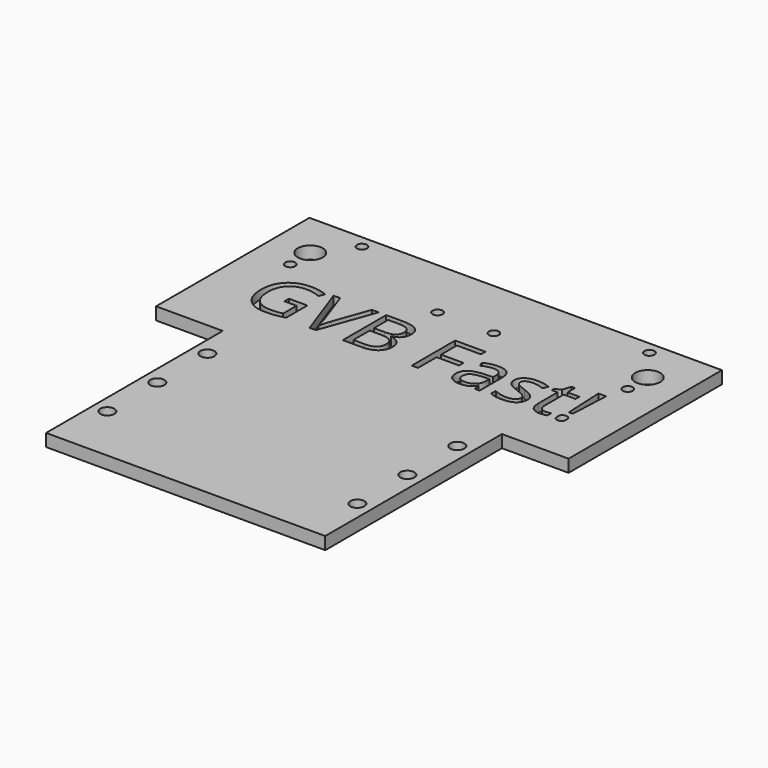
from build123d import *

# Parameters (mm, degrees)
F0_R         = 1.7
F0_R_2       = 1.2
F0_R_3       = 3
F1_DEPTH     = 3
F3_TEXT_SIZE = 18.2238832532
F4_DEPTH     = 2


# Not quite as in the source:
# - Text() gives the source's letters only with a copy of the font that has no kerning and outlines rounded to 1/6400 em; it was checked with that copy


with BuildPart() as f1:
    # F0 (on Top) → F1 (new body)
    with BuildSketch(Plane.XY):
        Polygon((0, 52.7634354346), (-49.5, 52.7634354346), (-49.5, 6.7634354346), (-33.5, 6.7634354346), (-33.5, -46.2365645654), (0, -46.2365645654), (33.5, -46.2365645654), (33.5, 6.7634354346), (49.5, 6.7634354346), (49.5, 52.7634354346), align=None)
        with Locations((-30, -32.2365645654)):
            Circle(F0_R, mode=Mode.SUBTRACT)
        with Locations((-30, -17.2365645654)):
            Circle(F0_R, mode=Mode.SUBTRACT)
        with Locations((-30, -2.2365645654)):
            Circle(F0_R, mode=Mode.SUBTRACT)
        with Locations((30, -32.2365645654)):
            Circle(F0_R, mode=Mode.SUBTRACT)
        with Locations((30, -17.2365645654)):
            Circle(F0_R, mode=Mode.SUBTRACT)
        with Locations((30, -2.2365645654)):
            Circle(F0_R, mode=Mode.SUBTRACT)
        with Locations((-40.5, 35.7634354346)):
            Circle(F0_R_2, mode=Mode.SUBTRACT)
        with Locations((-40.5, 41.7634354346)):
            Circle(F0_R_3, mode=Mode.SUBTRACT)
        with Locations((-34.5, 49.7634354346)):
            Circle(F0_R_2, mode=Mode.SUBTRACT)
        with Locations((-6.75, 37.7634354346)):
            Circle(F0_R_2, mode=Mode.SUBTRACT)
        with Locations((6.75, 37.7634354346)):
            Circle(F0_R_2, mode=Mode.SUBTRACT)
        with Locations((40.5, 35.7634354346)):
            Circle(F0_R_2, mode=Mode.SUBTRACT)
        with Locations((34.5, 49.7634354346)):
            Circle(F0_R_2, mode=Mode.SUBTRACT)
        with Locations((40.5, 41.7634354346)):
            Circle(F0_R_3, mode=Mode.SUBTRACT)
    extrude(amount=F1_DEPTH)

    # F3 (on face) + F0 (on Top) → F4 (cut)
    with BuildSketch(Plane.XY.offset(3)):
        with Locations((-39.5, 17.9082151303)):
            Text('GVB Fast!', F3_TEXT_SIZE, font='Open Sans', text_align=(TextAlign.LEFT, TextAlign.BOTTOM))
    with BuildSketch(Plane.XY):
        Polygon((0, 52.7634354346), (-49.5, 52.7634354346), (-49.5, 6.7634354346), (-33.5, 6.7634354346), (-33.5, -46.2365645654), (0, -46.2365645654), (33.5, -46.2365645654), (33.5, 6.7634354346), (49.5, 6.7634354346), (49.5, 52.7634354346), align=None)
        with Locations((-30, -32.2365645654)):
            Circle(F0_R, mode=Mode.SUBTRACT)
        with Locations((-30, -17.2365645654)):
            Circle(F0_R, mode=Mode.SUBTRACT)
        with Locations((-30, -2.2365645654)):
            Circle(F0_R, mode=Mode.SUBTRACT)
        with Locations((30, -32.2365645654)):
            Circle(F0_R, mode=Mode.SUBTRACT)
        with Locations((30, -17.2365645654)):
            Circle(F0_R, mode=Mode.SUBTRACT)
        with Locations((30, -2.2365645654)):
            Circle(F0_R, mode=Mode.SUBTRACT)
        with Locations((-40.5, 35.7634354346)):
            Circle(F0_R_2, mode=Mode.SUBTRACT)
        with Locations((-40.5, 41.7634354346)):
            Circle(F0_R_3, mode=Mode.SUBTRACT)
        with Locations((-34.5, 49.7634354346)):
            Circle(F0_R_2, mode=Mode.SUBTRACT)
        with Locations((-6.75, 37.7634354346)):
            Circle(F0_R_2, mode=Mode.SUBTRACT)
        with Locations((6.75, 37.7634354346)):
            Circle(F0_R_2, mode=Mode.SUBTRACT)
        with Locations((40.5, 35.7634354346)):
            Circle(F0_R_2, mode=Mode.SUBTRACT)
        with Locations((34.5, 49.7634354346)):
            Circle(F0_R_2, mode=Mode.SUBTRACT)
        with Locations((40.5, 41.7634354346)):
            Circle(F0_R_3, mode=Mode.SUBTRACT)
    extrude(amount=-F4_DEPTH, mode=Mode.SUBTRACT)


solid = f1.part
